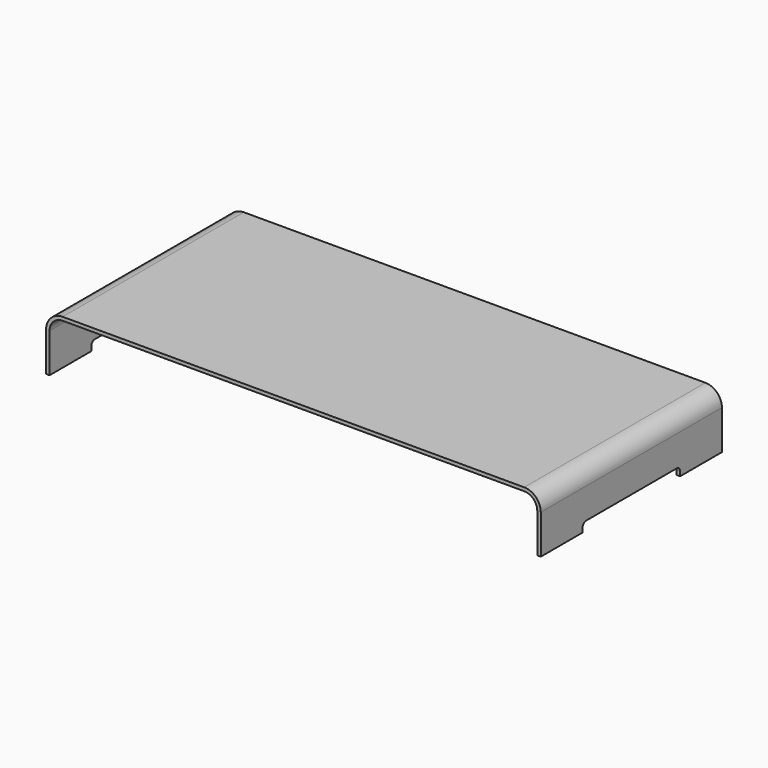
from build123d import *

# Parameters (mm, degrees)
F1_DEPTH = 130
F3_DEPTH = 600


with BuildPart() as f1:
    # F0 (on Front) → F1 (new body, symmetric)
    with BuildSketch(Plane.XZ):
        with BuildLine():
            Line((-250.1273464697, -45), (-246.1273464697, -45))
            Line((-246.1273464697, -45), (-246.1273464697, 0))
            ThreePointArc((-246.1273464697, 0), (-241.7339481875, 10.6066017178), (-231.1273464697, 15))
            Line((-231.1273464697, 15), (298.8726535303, 15))
            ThreePointArc((298.8726535303, 15), (309.4792552481, 10.6066017178), (313.8726535303, 0))
            Line((313.8726535303, 0), (313.8726535303, -45))
            Line((313.8726535303, -45), (317.8726535303, -45))
            Line((317.8726535303, -45), (317.8726535303, 0))
            ThreePointArc((317.8726535303, 0), (312.3076823729, 13.4350288425), (298.8726535303, 19))
            Line((298.8726535303, 19), (-231.1273464697, 19))
            ThreePointArc((-231.1273464697, 19), (-244.5623753122, 13.4350288425), (-250.1273464697, 0))
            Line((-250.1273464697, 0), (-250.1273464697, -45))
        make_face()
    extrude(amount=F1_DEPTH, both=True)

    # F2 (on face) → F3 (cut)
    with BuildSketch(Plane.YZ.offset(317.8726535303)):
        with BuildLine():
            Line((-70, -45), (70, -45))
            Line((70, -45), (70, -40))
            ThreePointArc((70, -40), (68.5355339059, -36.4644660941), (65, -35))
            Line((65, -35), (-65, -35))
            ThreePointArc((-65, -35), (-68.5355339059, -36.4644660941), (-70, -40))
            Line((-70, -40), (-70, -45))
        make_face()
    extrude(amount=-F3_DEPTH, mode=Mode.SUBTRACT)


solid = f1.part
